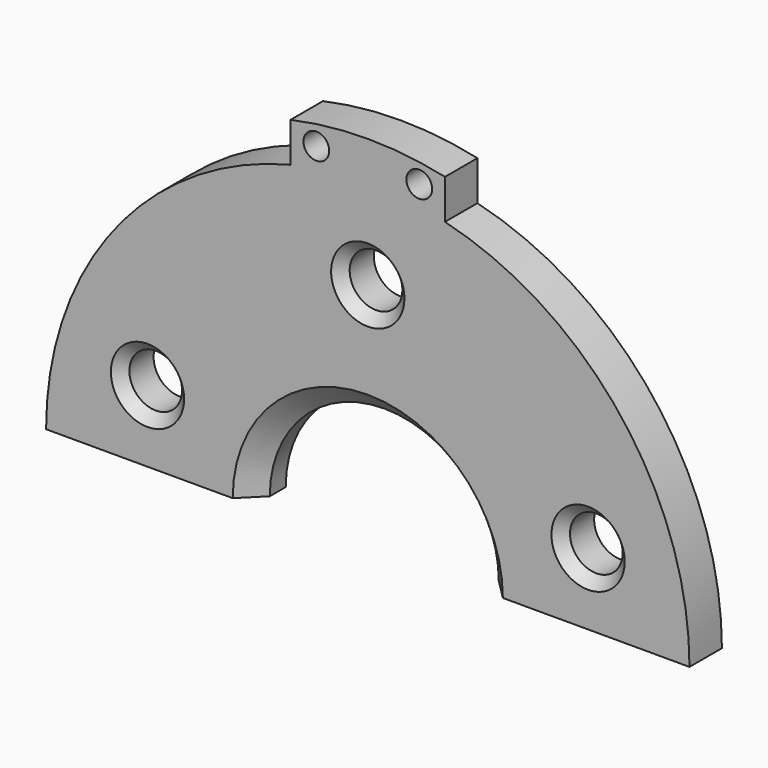
from build123d import *

# Parameters (mm, degrees)
F2_R     = 6.5
F2_R_2   = 3.175
F3_DEPTH = 10
F0_SIZE  = 5.08
F1_SIZE  = 2.54


# Not quite as in the source:
# - a feature names something its author has since deleted; it is built from what else it names


with BuildPart() as f3:
    # F2 (on Front) → F3 (new body)
    with BuildSketch(Plane.XZ):
        with BuildLine():
            Line((-19.05, 86.834944003), (-19.05, 77.0550979819))
            ThreePointArc((-19.05, 77.0550979819), (-62.4999375, 48.9300361486), (-79.375, 0))
            Line((-79.375, 0), (-28.25, 0))
            ThreePointArc((-28.25, 0), (0, 28.25), (28.25, 0))
            Line((28.25, 0), (79.375, 0))
            ThreePointArc((79.375, 0), (62.4999375, 48.9300361486), (19.05, 77.0550979819))
            Line((19.05, 77.0550979819), (19.05, 86.834944003))
            ThreePointArc((19.05, 86.834944003), (0, 88.9), (-19.05, 86.834944003))
        make_face()
        with Locations((-54.3528799063, 17.6603212285)):
            Circle(F2_R, mode=Mode.SUBTRACT)
        with Locations((54.3528799063, 17.6603212285)):
            Circle(F2_R, mode=Mode.SUBTRACT)
        with Locations((-12.7, 83.1734867987)):
            Circle(F2_R_2, mode=Mode.SUBTRACT)
        with Locations((0, 57.15)):
            Circle(F2_R, mode=Mode.SUBTRACT)
        with Locations((12.7, 83.1734867987)):
            Circle(F2_R_2, mode=Mode.SUBTRACT)
    extrude(amount=F3_DEPTH)

    # F0
    f0_edges = [f3.edges().sort_by_distance(p)[0] for p in [
        (0, -10, 28.25),
    ]]
    chamfer(f0_edges, length=F0_SIZE)

    # F1
    f1_edges = [f3.edges().sort_by_distance(p)[0] for p in [
        (-6.5, -10, 57.15),
        (-60.85288, -10, 17.660321),
        (47.85288, -10, 17.660321),
    ]]
    chamfer(f1_edges, length=F1_SIZE)


solid = f3.part
